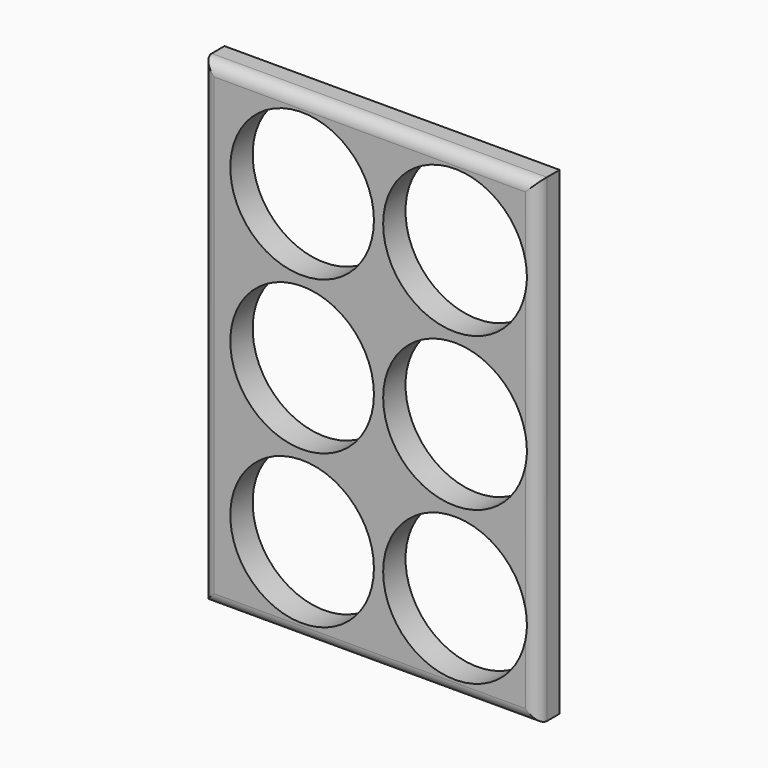
from build123d import *

# Parameters (mm, degrees)
F0_W        = 4
F0_H        = 120
F0_R        = 18
F1_DEPTH    = 7
F2_T1_DEPTH = 135
F2_T3_DEPTH = 99
F3_T        = -1


# Not quite as in the source:
# - a fillet or chamfer that OpenCascade refuses, or shapes differently, is made with other operations: its cross-section is extruded or revolved along the edge and cut away or added


with BuildPart() as f1:
    # F0 (on Front) → F1 (new body)
    with BuildSketch(Plane.XZ):
        with Locations((-42.8557436466, 2.7328292441)):
            Rectangle(F0_W, F0_H)
        Polygon((-0.6441245232, 2.7376232945), (-0.6441245232, 62.7328292441), (-40.8557436466, 62.7328292441), (-40.8557436466, -57.2671707559), (-0.6441245232, -57.2671707559), align=None)
        with Locations((-19.8015584055, -35.636439333)):
            Circle(F0_R, mode=Mode.SUBTRACT)
        with Locations((-19.8015584055, 2.7376232945)):
            Circle(F0_R, mode=Mode.SUBTRACT)
        with Locations((-19.8015584055, 41.1116859221)):
            Circle(F0_R, mode=Mode.SUBTRACT)
        Polygon((39.1442563534, -57.2671707559), (39.1442563534, 62.7328292441), (-0.6441245232, 62.7328292441), (-0.6441245232, 2.7376232945), (-0.6441245232, -57.2671707559), align=None)
        with Locations((18.5133093592, -35.636439333)):
            Circle(F0_R, mode=Mode.SUBTRACT)
        with Locations((18.5133093592, 2.7376232945)):
            Circle(F0_R, mode=Mode.SUBTRACT)
        with Locations((18.5133093592, 41.1116859221)):
            Circle(F0_R, mode=Mode.SUBTRACT)
    extrude(amount=F1_DEPTH)

    # F2: fillet of radius 3 on 4 edges, made by hand

    # F2_s2 → F2_t1 (cut)
    with BuildSketch(Plane.XY.offset(-64.7671707559)):
        with BuildLine():
            ThreePointArc((-44.8557436466, -4), (-43.9770639902, -6.1213203436), (-41.8557436466, -7))
            Line((-41.8557436466, -7), (-44.8557436466, -7))
            Line((-44.8557436466, -7), (-44.8557436466, -4))
        make_face()
        with BuildLine():
            ThreePointArc((39.1442563534, -4), (38.2655766969, -6.1213203436), (36.1442563534, -7))
            Line((36.1442563534, -7), (39.1442563534, -7))
            Line((39.1442563534, -7), (39.1442563534, -4))
        make_face()
    extrude(amount=F2_T1_DEPTH, mode=Mode.SUBTRACT)

    # F2_s4 → F2_t3 (cut)
    with BuildSketch(Plane.YZ.offset(-52.3557436466)):
        with BuildLine():
            ThreePointArc((-4, -57.2671707559), (-6.1213203436, -56.3884910995), (-7, -54.2671707559))
            Line((-7, -54.2671707559), (-7, -57.2671707559))
            Line((-7, -57.2671707559), (-4, -57.2671707559))
        make_face()
        with BuildLine():
            ThreePointArc((-4, 62.7328292441), (-6.1213203436, 61.8541495876), (-7, 59.7328292441))
            Line((-7, 59.7328292441), (-7, 62.7328292441))
            Line((-7, 62.7328292441), (-4, 62.7328292441))
        make_face()
    extrude(amount=F2_T3_DEPTH, mode=Mode.SUBTRACT)

    # F3
    f3_openings = [f1.faces().sort_by_distance(p)[0] for p in [
        (-43.390957, 0, 2.732829),
    ]]
    offset(amount=F3_T, openings=f3_openings)


solid = f1.part
